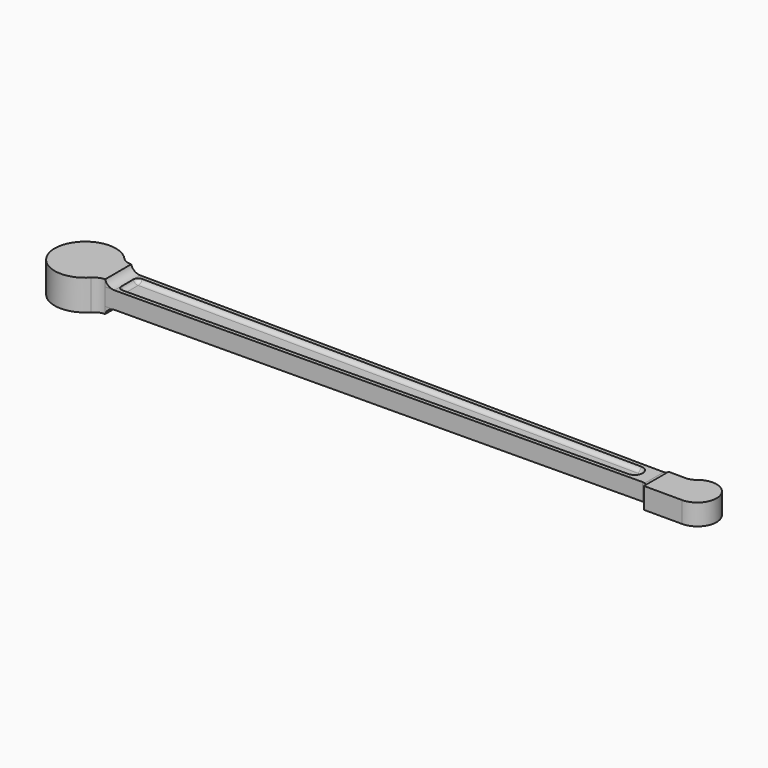
from build123d import *

# Parameters (mm, degrees)
F1_DEPTH     = 3.571875
F2_DEPTH     = 6.35
F3_DEPTH     = 4.365625
F4_T4_DEPTH  = 32.5377920371
F4_T10_DEPTH = 32.5377920371
F5_T4_DEPTH  = 22.8781953851
F5_S7_R      = 3
F5_T8_DEPTH  = 13
F5_T12_DEPTH = 22.8781953851
F5_S15_R     = 3
F5_T16_DEPTH = 13
F7_DEPTH     = 1.5875
F8_T1_DEPTH  = 208.4599958687
F8_T3_DEPTH  = 208.5127323296
F8_T5_DEPTH  = 6.2192364317
F8_T8_ANGLE  = 90
F8_T10_ANGLE = 179.0283359547
F8_T12_ANGLE = 90.9716640453


# Not quite as in the source:
# - a fillet or chamfer that OpenCascade refuses, or shapes differently, is made with other operations: its cross-section is extruded or revolved along the edge and cut away or added


with BuildPart() as f1:
    # F0 (on Top) → F1 (new body, symmetric)
    with BuildSketch(Plane.XY):
        with BuildLine():
            ThreePointArc((-113.3683072515, 6.746875), (-115.7345796972, 7.2550843623), (-117.7075605328, 8.656822093))
            ThreePointArc((-117.7075605328, 8.656822093), (-139.7, 0), (-117.7075605328, -8.656822093))
            ThreePointArc((-117.7075605328, -8.656822093), (-115.7345796972, -7.2550843623), (-113.3683072515, -6.746875))
            Line((-113.3683072515, -6.746875), (-113.3683072515, 6.746875))
        make_face()
        with BuildLine():
            Line((111.125, 4.8432679198), (-113.3683072515, 6.746875))
            Line((-113.3683072515, 6.746875), (-113.3683072515, -6.746875))
            Line((-113.3683072515, -6.746875), (108.0995621996, -4.8689223364))
            ThreePointArc((108.0995621996, -4.8689223364), (110.2373075769, -5.7385195078), (111.125, -7.8688144875))
            Line((111.125, -7.8688144875), (111.125, 4.8432679198))
        make_face()
        with BuildLine():
            Line((118.1193570388, 4.7839587683), (111.125, 4.8432679198))
            Line((111.125, 4.8432679198), (111.125, -7.8688144875))
            Line((111.125, -7.8688144875), (111.125, -7.9375))
            Line((111.125, -7.9375), (127, -7.9375))
            ThreePointArc((127, -7.9375), (134.4750044007, 2.6698718057), (121.9713880952, 6.141414215))
            ThreePointArc((121.9713880952, 6.141414215), (120.1644294879, 5.1248404445), (118.1193570388, 4.7839587683))
        make_face()
    extrude(amount=F1_DEPTH, both=True)

    # F0 (on Top) → F2 (join, symmetric)
    with BuildSketch(Plane.XY):
        with BuildLine():
            ThreePointArc((-113.3683072515, 6.746875), (-115.7345796972, 7.2550843623), (-117.7075605328, 8.656822093))
            ThreePointArc((-117.7075605328, 8.656822093), (-139.7, 0), (-117.7075605328, -8.656822093))
            ThreePointArc((-117.7075605328, -8.656822093), (-115.7345796972, -7.2550843623), (-113.3683072515, -6.746875))
            Line((-113.3683072515, -6.746875), (-113.3683072515, 6.746875))
        make_face()
    extrude(amount=F2_DEPTH, both=True)

    # F0 (on Top) → F3 (join, symmetric)
    with BuildSketch(Plane.XY):
        with BuildLine():
            Line((118.1193570388, 4.7839587683), (111.125, 4.8432679198))
            Line((111.125, 4.8432679198), (111.125, -7.8688144875))
            Line((111.125, -7.8688144875), (111.125, -7.9375))
            Line((111.125, -7.9375), (127, -7.9375))
            ThreePointArc((127, -7.9375), (134.4750044007, 2.6698718057), (121.9713880952, 6.141414215))
            ThreePointArc((121.9713880952, 6.141414215), (120.1644294879, 5.1248404445), (118.1193570388, 4.7839587683))
        make_face()
    extrude(amount=F3_DEPTH, both=True)

    # F4: fillet of radius 4 on 2 edges, made by hand


with BuildPart() as f4_tool2:
    # F4_s3 → F4_t4 (new body)
    with BuildSketch(Plane.XZ.offset(16.2688960185)):
        with BuildLine():
            ThreePointArc((-109.5594988441, 3.571875), (-111.9166687573, 4.3401958699), (-113.3683072515, 6.35))
            Line((-113.3683072515, 6.35), (-113.3683072515, 3.571875))
            Line((-113.3683072515, 3.571875), (-109.5594988441, 3.571875))
        make_face()
    extrude(amount=-F4_T4_DEPTH)

    split(bisect_by=Plane(origin=(0.0490555459, 5.7851443476, 0), x_dir=(0, 0, 1), z_dir=(-0.0084792668, -0.9999640504, 0)), keep=Keep.TOP)

    split(bisect_by=Plane(origin=(0.0490555459, -5.7851443476, 0), x_dir=(0, 0, 1), z_dir=(-0.0084792668, 0.9999640504, 0)), keep=Keep.TOP)


with BuildPart() as f1_1:
    add(f1.part)

    # F4_t1: union F4_tool2
    add(f4_tool2.part)


with BuildPart() as f4_tool8:
    # F4_s9 → F4_t10 (new body)
    with BuildSketch(Plane.XZ.offset(16.2688960185)):
        with BuildLine():
            ThreePointArc((-113.3683072515, -6.35), (-111.9166687573, -4.3401958699), (-109.5594988441, -3.571875))
            Line((-109.5594988441, -3.571875), (-113.3683072515, -3.571875))
            Line((-113.3683072515, -3.571875), (-113.3683072515, -6.35))
        make_face()
    extrude(amount=-F4_T10_DEPTH)

    split(bisect_by=Plane(origin=(0.0490555459, 5.7851443476, 0), x_dir=(0, 0, 1), z_dir=(-0.0084792668, -0.9999640504, 0)), keep=Keep.TOP)

    split(bisect_by=Plane(origin=(0.0490555459, -5.7851443476, 0), x_dir=(0, 0, 1), z_dir=(-0.0084792668, 0.9999640504, 0)), keep=Keep.TOP)


with BuildPart() as f1_2:
    add(f1_1.part)

    # F4_t7: union F4_tool8
    add(f4_tool8.part)

    # F5: fillet of radius 3 on 2 edges, made by hand


with BuildPart() as f5_tool2:
    # F5_s3 → F5_t4 (new body)
    with BuildSketch(Plane.XZ.offset(-9.9263244087)):
        with BuildLine():
            ThreePointArc((111.1252710091, -4.3653307993), (110.1832561552, -3.7769740577), (109.0917774438, -3.571475))
            Line((109.0917774438, -3.571475), (109.0917774438, -3.2713384315))
            ThreePointArc((109.0917774438, -3.2713384315), (110.1083887219, -3.2717384315), (111.125, -3.2717384315))
            Line((111.125, -3.2717384315), (111.4251365685, -3.571875))
            ThreePointArc((111.4251365685, -3.571875), (111.4251365685, -3.9686028996), (111.3286203656, -4.1445798107))
            Line((111.3286203656, -4.1445798107), (111.1252710091, -4.3653307993))
        make_face()
    extrude(amount=F5_T4_DEPTH)

    split(bisect_by=Plane(origin=(0.0490555459, 5.7851443476, 0), x_dir=(0, 0, 1), z_dir=(-0.0084792668, -0.9999640504, 0)), keep=Keep.TOP)

    split(bisect_by=Plane.XZ.offset(7.9375), keep=Keep.BOTTOM)

    # F5_s7 → F5_t8 (cut, symmetric)
    with BuildSketch(Plane.XY.offset(-3.8)):
        with Locations((108.125, -7.8688144875)):
            Circle(F5_S7_R)
    extrude(amount=F5_T8_DEPTH, both=True, mode=Mode.SUBTRACT)


with BuildPart() as f1_3:
    add(f1_2.part)

    # F5_t1: union F5_tool2
    add(f5_tool2.part)


with BuildPart() as f5_tool10:
    # F5_s11 → F5_t12 (new body)
    with BuildSketch(Plane.XZ.offset(-9.9263244087)):
        with BuildLine():
            ThreePointArc((111.1252710091, 4.3653307993), (110.1832561552, 3.7769740577), (109.0917774438, 3.571475))
            Line((109.0917774438, 3.571475), (109.0917774438, 3.2713384315))
            ThreePointArc((109.0917774438, 3.2713384315), (110.1083887219, 3.2717384315), (111.125, 3.2717384315))
            Line((111.125, 3.2717384315), (111.4251365685, 3.571875))
            ThreePointArc((111.4251365685, 3.571875), (111.4251365685, 3.9686028996), (111.3286203656, 4.1445798107))
            Line((111.3286203656, 4.1445798107), (111.1252710091, 4.3653307993))
        make_face()
    extrude(amount=F5_T12_DEPTH)

    split(bisect_by=Plane(origin=(0.0490555459, 5.7851443476, 0), x_dir=(0, 0, 1), z_dir=(-0.0084792668, -0.9999640504, 0)), keep=Keep.TOP)

    split(bisect_by=Plane.XZ.offset(7.9375), keep=Keep.BOTTOM)

    # F5_s15 → F5_t16 (cut, symmetric)
    with BuildSketch(Plane.XY.offset(3.8)):
        with Locations((108.125, -7.8688144875)):
            Circle(F5_S15_R)
    extrude(amount=F5_T16_DEPTH, both=True, mode=Mode.SUBTRACT)


with BuildPart() as f1_4:
    add(f1_3.part)

    # F5_t9: union F5_tool10
    add(f5_tool10.part)

    # F6 (on face) → F7 (cut)
    with BuildSketch(Plane.XY.offset(3.571875)):
        with BuildLine():
            Line((-107.4591662774, -5.1092109437), (100.9933355318, -3.3416230224))
            ThreePointArc((100.9933355318, -3.3416230224), (104.3067431568, 0), (100.9933355318, 3.3416230224))
            Line((100.9933355318, 3.3416230224), (-107.5119008424, 5.1096581102))
            ThreePointArc((-107.5119008424, 5.1096581102), (-108.9430729384, 4.5239435719), (-109.5287874768, 3.0927714759))
            Line((-109.5287874768, 3.0927714759), (-109.4760529118, -3.1262413766))
            ThreePointArc((-109.4760529118, -3.1262413766), (-108.8782960389, -4.535437059), (-107.4591662774, -5.1092109437))
        make_face()
    extrude(amount=-F7_DEPTH, mode=Mode.SUBTRACT)

    # F8: fillet of radius 2 on 1 edges, made by hand

    # F8_s2 → F8_t1 (join)
    with BuildSketch(Plane(origin=(-107.4947609873, -0.9115095261, 0), x_dir=(0, 0, 1), z_dir=(0.9999640504, 0.0084792668, 0))):
        with BuildLine():
            ThreePointArc((3.571875, 4.1978523289), (2.4311525433, 3.5008139871), (1.984375, 2.2408536702))
            Line((1.984375, 2.2408536702), (1.984375, 4.1978523289))
            Line((1.984375, 4.1978523289), (3.571875, 4.1978523289))
        make_face()
    extrude(amount=F8_T1_DEPTH)

    # F8_s4 → F8_t3 (join)
    with BuildSketch(Plane(origin=(100.9577408219, -0.8560783953, 0), x_dir=(0, 0, 1), z_dir=(-0.9999640504, 0.0084792668, 0))):
        with BuildLine():
            ThreePointArc((3.571875, 4.1978523289), (2.4311525433, 3.5008139871), (1.984375, 2.2408536702))
            Line((1.984375, 2.2408536702), (1.984375, 4.1978523289))
            Line((1.984375, 4.1978523289), (3.571875, 4.1978523289))
        make_face()
    extrude(amount=F8_T3_DEPTH)

    # F8_s6 → F8_t5 (join)
    with BuildSketch(Plane(origin=(-0.0340983887, 4.0212395356, 0), x_dir=(0, 0, 1), z_dir=(0.0084792668, -0.9999640504, 0))):
        with BuildLine():
            ThreePointArc((3.571875, 109.498625523), (2.4311525433, 108.8015871812), (1.984375, 107.5416268643))
            Line((1.984375, 107.5416268643), (1.984375, 109.498625523))
            Line((1.984375, 109.498625523), (3.571875, 109.498625523))
        make_face()
    extrude(amount=F8_T5_DEPTH)

    # F8_s7 → F8_t8 (revolve)
    with BuildSketch(Plane(origin=(0.0186361763, -2.1977733169, 0), x_dir=(0, 0, 1), z_dir=(-0.0084792668, 0.9999640504, 0))):
        with BuildLine():
            ThreePointArc((3.571875, -109.498625523), (2.4311525433, -108.8015871812), (1.984375, -107.5416268643))
            Line((1.984375, -107.5416268643), (1.984375, -109.498625523))
            Line((1.984375, -109.498625523), (3.571875, -109.498625523))
        make_face()
    revolve(axis=Axis((-107.476124811, -3.109282843, 1.984375), (0, 0, 1)), revolution_arc=F8_T8_ANGLE)

    # F8_s9 → F8_t10 (revolve)
    with BuildSketch(Plane(origin=(100.9577408219, 0.8560783953, 0), x_dir=(0, 0, 1), z_dir=(-0.9999640504, -0.0084792668, 0))):
        with BuildLine():
            ThreePointArc((3.571875, -4.1978523289), (2.4311525433, -3.5008139871), (1.984375, -2.2408536702))
            Line((1.984375, -2.2408536702), (1.984375, -4.1978523289))
            Line((1.984375, -4.1978523289), (3.571875, -4.1978523289))
        make_face()
    revolve(axis=Axis((100.965, 0, 1.984375), (0, 0, 1)), revolution_arc=F8_T10_ANGLE)

    # F8_s11 → F8_t12 (revolve)
    with BuildSketch(Plane(origin=(-107.5474955523, 0.9119566926, 0), x_dir=(0, 0, 1), z_dir=(0.9999640504, -0.0084792668, 0))):
        with BuildLine():
            ThreePointArc((3.571875, -4.1978523289), (2.4311525433, -3.5008139871), (1.984375, -2.2408536702))
            Line((1.984375, -2.2408536702), (1.984375, -4.1978523289))
            Line((1.984375, -4.1978523289), (3.571875, -4.1978523289))
        make_face()
    revolve(axis=Axis((-107.528859376, 3.1097300095, 1.984375), (0, 0, 1)), revolution_arc=F8_T12_ANGLE)


solid = f1_4.part
